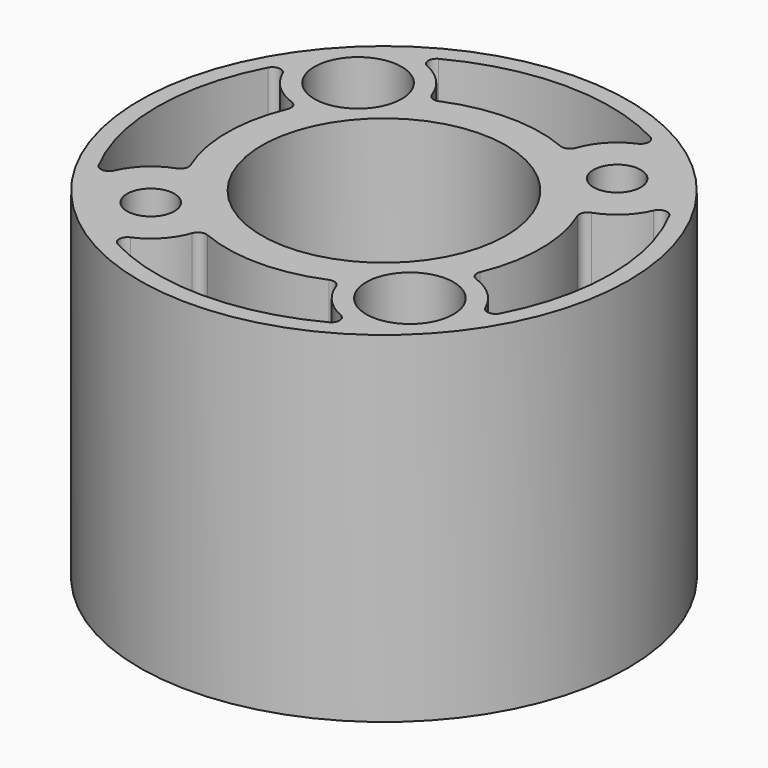
from build123d import *

# Parameters (mm, degrees)
F0_R            = 22.225
F0_R_2          = 2.15265
F0_R_3          = 11.1125
F1_DEPTH        = 31
F3_DEPTH        = 31
F3_COPIES_COUNT = 4
F4_R            = 0.762
F7_R            = 3.96875
F7_R_2          = 2.15265
F10_DEPTH       = 27.825
F6_R            = 3.96875
F6_R_2          = 2.15265
F11_DEPTH       = 27.825


# Not quite as in the source:
# - a feature of the source that left no trace in its solid (it failed there, or was rolled back) is left out
# - a pattern or mirror of a feature is missing from the dataset's text; its kind, count and spacing are read off the source's solid


with BuildPart() as f1:
    # F0 (on Top) → F1 (new body)
    with BuildSketch(Plane.XY):
        Circle(F0_R)
        with Locations((-11.7865861589, -11.7865861589)):
            Circle(F0_R_2, mode=Mode.SUBTRACT)
        with Locations((11.7865861589, -11.7865861589)):
            Circle(F0_R_2, mode=Mode.SUBTRACT)
        with Locations((-11.7865861589, 11.7865861589)):
            Circle(F0_R_2, mode=Mode.SUBTRACT)
        Circle(F0_R_3, mode=Mode.SUBTRACT)
        with Locations((11.7865861589, 11.7865861589)):
            Circle(F0_R_2, mode=Mode.SUBTRACT)
    extrude(amount=F1_DEPTH)

    # F2 (on face) → F3 (cut, through all)
    with BuildSketch(Plane(origin=(0, 0, 0), x_dir=(1, 0, 0), z_dir=(0, 0, -1))):
        with BuildLine():
            ThreePointArc((11.229543123, -17.3148424047), (8.0281867, -15.8788163052), (6.3255746232, -12.8109235396))
            ThreePointArc((6.3255746232, -12.8109235396), (0, -14.2875), (-6.3255746232, -12.8109235396))
            ThreePointArc((-6.3255746232, -12.8109235396), (-8.0281867, -15.8788163052), (-11.229543123, -17.3148424047))
            ThreePointArc((-11.229543123, -17.3148424047), (0, -20.6375), (11.229543123, -17.3148424047))
        make_face()
    f3 = extrude(amount=-F3_DEPTH, mode=Mode.SUBTRACT)

    # F3_copies: F3 ×4 about axis
    f3_copies_axis = Axis((0, 0, 0), (0, 0, 1))
    for i in range(1, F3_COPIES_COUNT):
        add(f3.rotate(f3_copies_axis, i * 360 / F3_COPIES_COUNT), mode=Mode.SUBTRACT)

    # F4
    f4_edges = [f1.edges().sort_by_distance(p)[0] for p in [
        (-6.325575, 12.810924, 15.5),
        (6.325575, 12.810924, 15.5),
        (11.229543, 17.314842, 15.5),
        (-11.229543, 17.314842, 15.5),
        (11.229543, -17.314842, 15.5),
        (-11.229543, -17.314842, 15.5),
        (6.325575, -12.810924, 15.5),
        (-6.325575, -12.810924, 15.5),
        (17.314842, 11.229543, 15.5),
        (17.314842, -11.229543, 15.5),
        (12.810924, 6.325575, 15.5),
        (12.810924, -6.325575, 15.5),
        (-17.314842, -11.229543, 15.5),
        (-17.314842, 11.229543, 15.5),
        (-12.810924, -6.325575, 15.5),
        (-12.810924, 6.325575, 15.5),
    ]]
    fillet(f4_edges, radius=F4_R)

    # F7 (on face) → F10 (cut, through all)
    with BuildSketch(Plane.XY.offset(31)):
        with Locations((-11.7865861589, 11.7865861589)):
            Circle(F7_R)
        with Locations((-11.7865861589, 11.7865861589)):
            Circle(F7_R_2, mode=Mode.SUBTRACT)
        with Locations((11.7865861589, -11.7865861589)):
            Circle(F7_R)
        with Locations((11.7865861589, -11.7865861589)):
            Circle(F7_R_2, mode=Mode.SUBTRACT)
    extrude(amount=-F10_DEPTH, mode=Mode.SUBTRACT)

    # F6 (on face) → F11 (cut, through all)
    with BuildSketch(Plane(origin=(0, 0, 0), x_dir=(1, 0, 0), z_dir=(0, 0, -1))):
        with Locations((11.7865861589, -11.7865861589)):
            Circle(F6_R)
        with Locations((11.7865861589, -11.7865861589)):
            Circle(F6_R_2, mode=Mode.SUBTRACT)
        with Locations((-11.7865861589, 11.7865861589)):
            Circle(F6_R)
        with Locations((-11.7865861589, 11.7865861589)):
            Circle(F6_R_2, mode=Mode.SUBTRACT)
    extrude(amount=-F11_DEPTH, mode=Mode.SUBTRACT)


solid = f1.part
